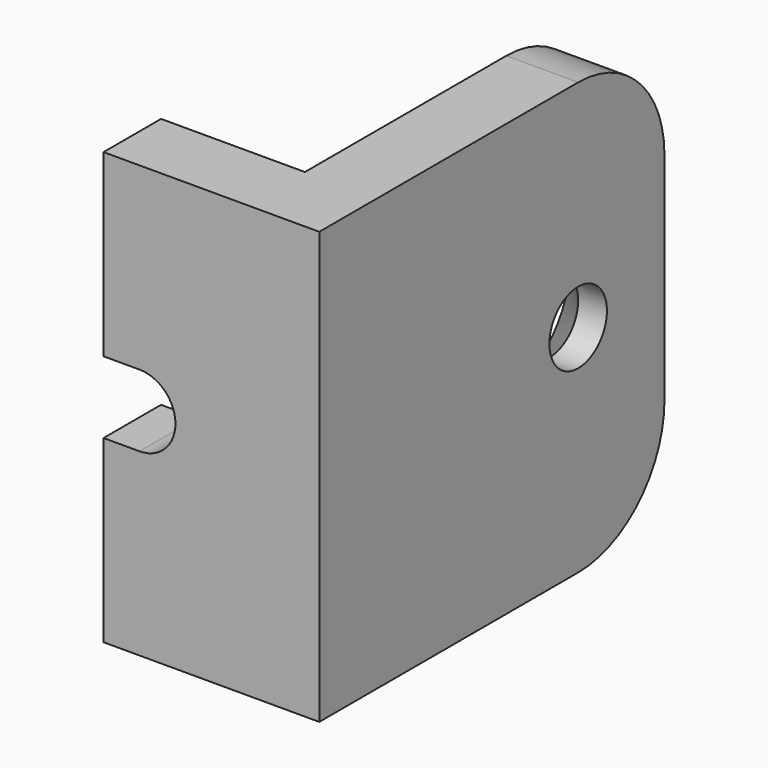
from build123d import *

# Parameters (mm, degrees)
F1_DEPTH = 76.2
F2_R     = 12.7
F3_DEPTH = 76.201
F5_DEPTH = 25.4
F8_DEPTH = 6.35
F9_R     = 38.1
F10_R    = 38.1
F11_SIZE = 15.24


# Not quite as in the source:
# - a pattern or mirror of a feature is missing from the dataset's text; its kind, count and spacing are read off the source's solid


with BuildPart() as f1:
    # F0 (on Top) → F1 (new body, symmetric)
    with BuildSketch(Plane.XY):
        Polygon((-76.2, 25.4), (-76.2, 0), (0, 0), (0, 152.4), (-25.4, 152.4), (-25.4, 25.4), align=None)
    extrude(amount=F1_DEPTH, both=True)

    # F2 (on face) → F3 (cut, through all)
    with BuildSketch(Plane.YZ):
        with Locations((114.3, 0)):
            Circle(F2_R)
    extrude(amount=-F3_DEPTH, mode=Mode.SUBTRACT)

    # F4 (on face) → F5 (cut)
    with BuildSketch(Plane.XZ):
        with BuildLine():
            ThreePointArc((-63.5, -12.7), (-50.8, 0), (-63.5, 12.7))
            Line((-63.5, 12.7), (-76.2, 12.7))
            Line((-76.2, 12.7), (-76.2, -12.7))
            Line((-76.2, -12.7), (-63.5, -12.7))
        make_face()
    extrude(amount=-F5_DEPTH, mode=Mode.SUBTRACT)

    # F7 (on offset) → F8 (join, symmetric)
    with BuildSketch(Plane.XY.offset(44.45)):
        Polygon((-50.8, 25.4), (-25.4, 25.4), (-25.4, 109.758593142), align=None)
    f8 = extrude(amount=F8_DEPTH, both=True)

    # F8_copies: F8 across plane
    add(f8.mirror(Plane(origin=(0, 0, 0), x_dir=(-1, 0, 0), z_dir=(0, 0, -1))))

    # F9
    f9_edges = [f1.edges().sort_by_distance(p)[0] for p in [
        (-12.7, 152.4, 76.2),
    ]]
    fillet(f9_edges, radius=F9_R)

    # F10
    f10_edges = [f1.edges().sort_by_distance(p)[0] for p in [
        (-12.7, 152.4, -76.2),
    ]]
    fillet(f10_edges, radius=F10_R)

    # F11
    f11_edges = [f1.edges().sort_by_distance(p)[0] for p in [
        (-25.4, 101.6, 0),
    ]]
    chamfer(f11_edges, length=F11_SIZE)


solid = f1.part
